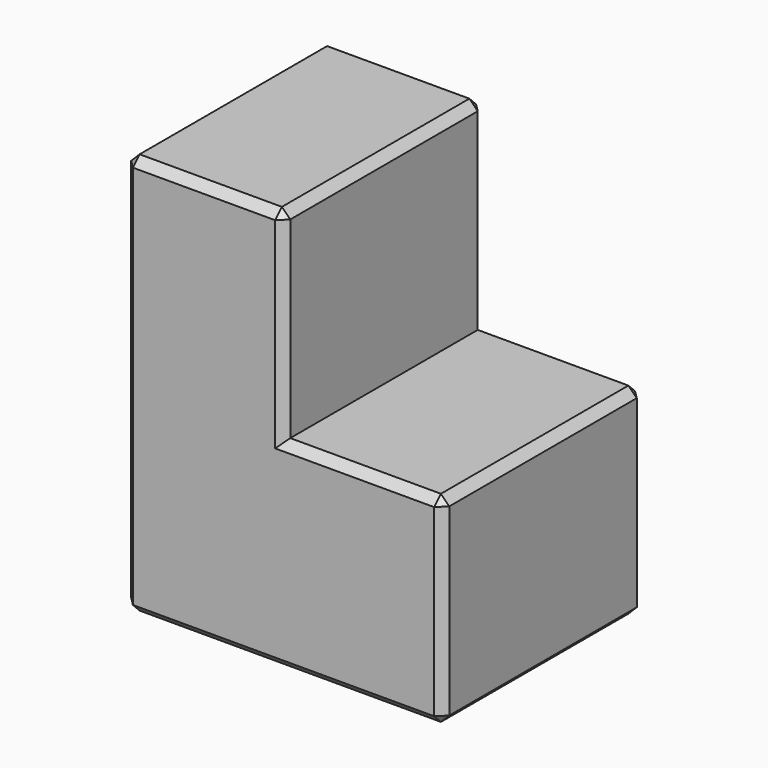
from build123d import *

# Parameters (mm, degrees)
F1_DEPTH = 30
F2_SIZE  = 1


# Not quite as in the source:
# - a feature names something its author has since deleted; it is built from what else it names


with BuildPart() as f1:
    # F0 (on Front) → F1 (new body)
    with BuildSketch(Plane.XZ):
        Polygon((19, 0), (0, 0), (0, 24), (-19, 24), (-19, -24), (19, -24), align=None)
    extrude(amount=F1_DEPTH)

    # F2
    f2_edges = [f1.edges().sort_by_distance(p)[0] for p in [
        (9.5, -30, 0),
        (0, -30, 12),
        (-9.5, -30, 24),
        (-19, -30, 0),
        (0, -30, -24),
        (19, -30, -12),
        (9.5, 0, 0),
        (0, 0, 12),
        (-9.5, 0, 24),
        (-19, 0, 0),
        (0, 0, -24),
        (19, 0, -12),
        (0, -15, 24),
        (-19, -15, 24),
        (-19, -15, -24),
        (19, -15, -24),
        (19, -15, 0),
    ]]
    chamfer(f2_edges, length=F2_SIZE)


solid = f1.part
